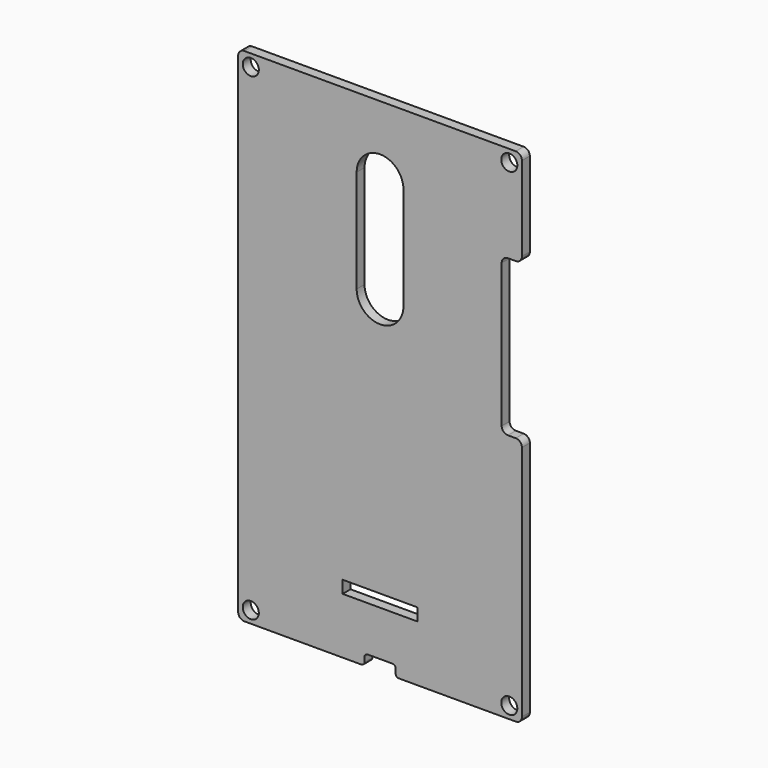
from build123d import *

# Parameters (mm, degrees)
F1_R     = 2.578
F1_W     = 24
F1_H     = 4
F2_DEPTH = 3.175
F3_R     = 2
F4_R     = 1


# Not quite as in the source:
# - a feature names something its author has since deleted; it is built from what else it names


with BuildPart() as f2:
    # F1 (on Front) → F2 (new body)
    with BuildSketch(Plane.XZ):
        Polygon((45.5, 49.5), (45.5, 80.5), (-45.5, 80.5), (-45.5, -80.5), (-5, -80.5), (-5, -77), (5, -77), (5, -80.5), (45.5, -80.5), (45.5, -0.5), (39, -0.5), (39, 49.5), align=None)
        with Locations((-41.4446451293, -76.6580848593)):
            Circle(F1_R, mode=Mode.SUBTRACT)
        with Locations((0, -60.5)):
            Rectangle(F1_W, F1_H, mode=Mode.SUBTRACT)
        with Locations((41.4446451293, -76.6580848593)):
            Circle(F1_R, mode=Mode.SUBTRACT)
        with Locations((-41.4446451293, 76.6580848593)):
            Circle(F1_R, mode=Mode.SUBTRACT)
        with BuildLine():
            ThreePointArc((-7.5, 58), (0, 65.5), (7.5, 58))
            Line((7.5, 58), (7.5, 25))
            ThreePointArc((7.5, 25), (0, 17.5), (-7.5, 25))
            Line((-7.5, 25), (-7.5, 58))
        make_face(mode=Mode.SUBTRACT)
        with Locations((41.4446451293, 76.6580848593)):
            Circle(F1_R, mode=Mode.SUBTRACT)
    extrude(amount=F2_DEPTH)

    # F3
    f3_edges = [f2.edges().sort_by_distance(p)[0] for p in [
        (-45.5, -1.5875, 80.5),
        (45.5, -1.5875, 80.5),
        (45.5, -1.5875, 49.5),
        (39, -1.5875, 49.5),
        (45.5, -1.5875, -0.5),
        (39, -1.5875, -0.5),
        (-45.5, -1.5875, -80.5),
        (45.5, -1.5875, -80.5),
    ]]
    fillet(f3_edges, radius=F3_R)

    # F4
    f4_edges = [f2.edges().sort_by_distance(p)[0] for p in [
        (5, -1.5875, -80.5),
        (5, -1.5875, -77),
        (-5, -1.5875, -77),
        (-5, -1.5875, -80.5),
    ]]
    fillet(f4_edges, radius=F4_R)


solid = f2.part
